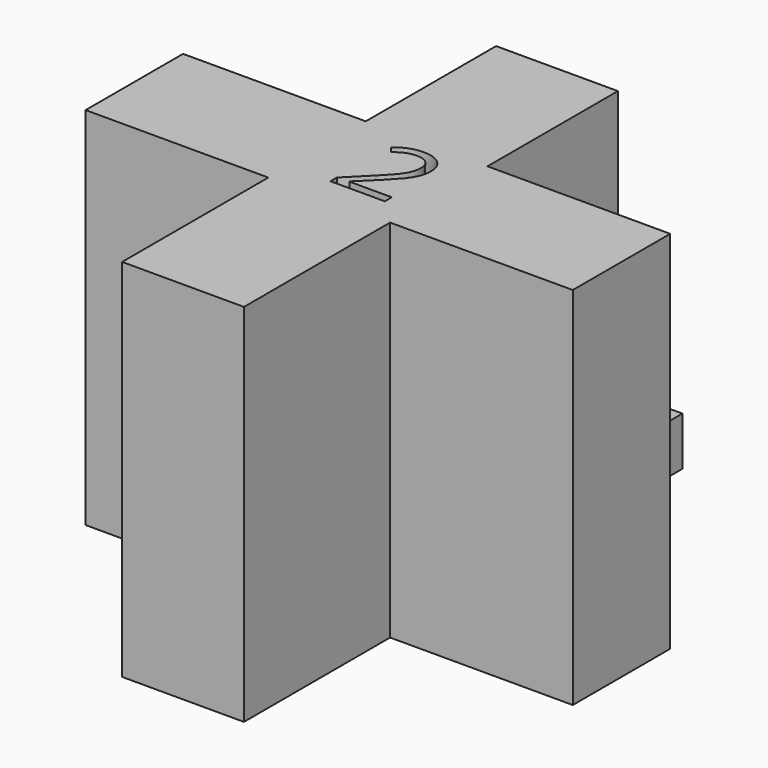
from build123d import *

# Parameters (mm, degrees)
F0_W         = 12.7
F0_H         = 57.15
F1_DEPTH     = 5.08
F2_W         = 50.8
F2_H         = 12.7
F3_DEPTH     = 38.1
F4_W         = 12.7
F4_H         = 48.7413735385
F5_DEPTH     = 33.02
F6_TEXT_SIZE = 12.0747026004
F7_DEPTH     = 2.54


# Not quite as in the source:
# - Text() gives the source's letters only with a copy of the font that has no kerning and outlines rounded to 1/6400 em; it was checked with that copy


with BuildPart() as f1:
    # F0 (on Top) → F1 (new body)
    with BuildSketch(Plane.XY):
        with Locations((-37.0165128261, 2.9978602284)):
            Rectangle(F0_W, F0_H)
    extrude(amount=F1_DEPTH)

    # F2 (on Top) → F3 (join)
    with BuildSketch(Plane.XY):
        with Locations((-37.0165128261, -0.1771397716)):
            Rectangle(F2_W, F2_H)
    extrude(amount=F3_DEPTH)

    # F4 (on face) → F5 (join)
    with BuildSketch(Plane.XY.offset(5.08)):
        with Locations((-37.0165128261, -1.2064530024)):
            Rectangle(F4_W, F4_H)
    extrude(amount=F5_DEPTH)

    # F6 (on face) → F7 (cut)
    with BuildSketch(Plane.XY.offset(38.1)):
        with Locations((-39.5974777639, -3.8714513648)):
            Text('2', F6_TEXT_SIZE, font='Open Sans', text_align=(TextAlign.LEFT, TextAlign.BOTTOM))
    extrude(amount=-F7_DEPTH, mode=Mode.SUBTRACT)


solid = f1.part
